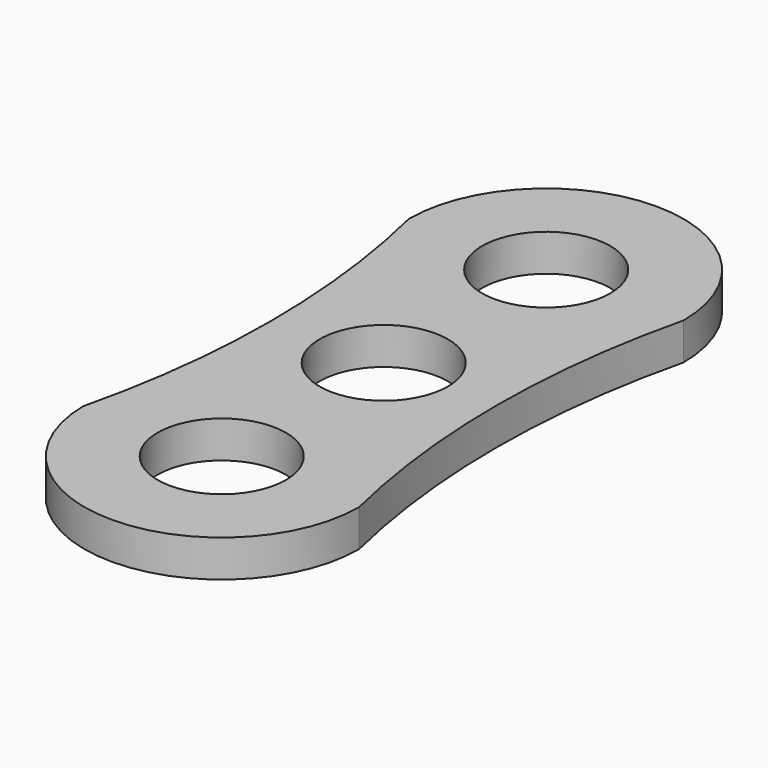
from build123d import *

# Parameters (mm, degrees)
F0_R     = 10.9982
F1_DEPTH = 6.35


# Not quite as in the source:
# - a feature names something its author has since deleted; it is built from what else it names


with BuildPart() as f1:
    # F0 (on Top) → F1 (new body)
    with BuildSketch(Plane.XY):
        with BuildLine():
            ThreePointArc((23.5712, -34.728333354), (19.5070052041, -0.0046640159), (23.674090089, 34.706808082))
            ThreePointArc((23.674090089, 34.706808082), (0.1039423202, 58.2769558508), (-23.4662054486, 34.706808082))
            ThreePointArc((-23.4662054486, 34.706808082), (-19.3723117522, -0.1418189062), (-23.569876554, -34.9781105903))
            ThreePointArc((-23.569876554, -34.9781105903), (0.1248903712, -58.2992024902), (23.5712, -34.728333354))
        make_face()
        with Locations((0, -34.728333354)):
            Circle(F0_R, mode=Mode.SUBTRACT)
        Circle(F0_R, mode=Mode.SUBTRACT)
        with Locations((0.1039423202, 34.706808082)):
            Circle(F0_R, mode=Mode.SUBTRACT)
    extrude(amount=F1_DEPTH)


solid = f1.part
